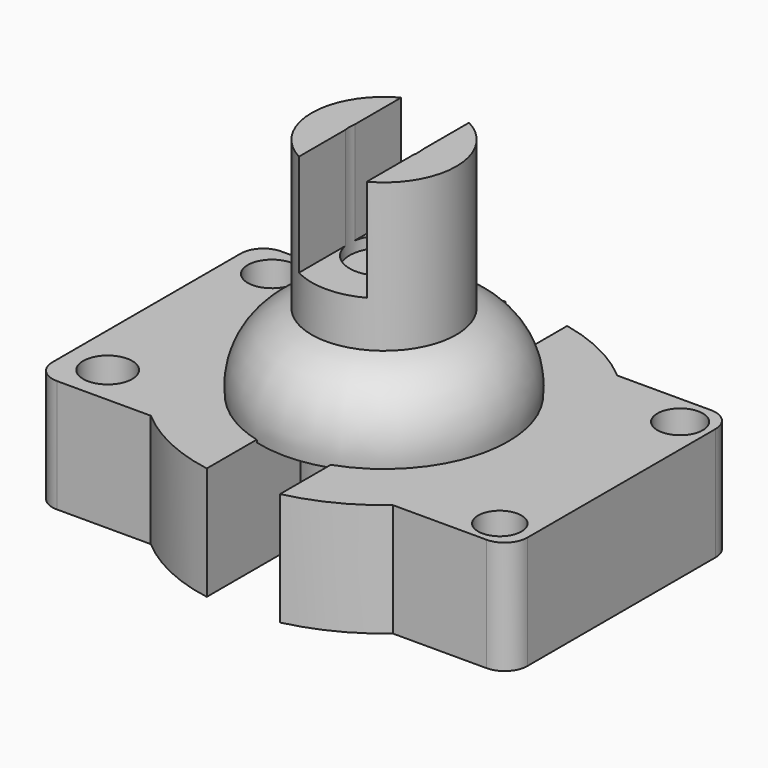
from build123d import *

# Parameters (mm, degrees)
F1_DEPTH       = 25.4
F2_R           = 5.4495134178
F2_R_2         = 5.5089125438
F3_DEPTH       = 25.4
F4_R           = 5.1025387704
F4_R_2         = 4.874193153
F5_DEPTH       = 25.4
F7_DEPTH       = 25.4
F9_DEPTH       = 25.4
F10_R          = 5.08
F15_R          = 7.7344411216
F16_DEPTH      = 25.4
F17_W          = 15.24
F17_H          = 33.801519665
F18_DEPTH      = 25.4
F18_DEPTH_BACK = 25.4


# Not quite as in the source:
# - a feature of the source that left no trace in its solid (it failed there, or was rolled back) is left out


with BuildPart() as f1:
    # F0 (on Top) → F1 (new body)
    with BuildSketch(Plane.XY):
        with BuildLine():
            Line((-53.3399991691, -31.5190926194), (-27.1817994649, -31.5190926194))
            ThreePointArc((-27.1817994649, -31.5190926194), (-41.6209493128, 0), (-27.1817994649, 31.5190926194))
            Line((-27.1817994649, 31.5190926194), (-53.3399991691, 31.5190926194))
            Line((-53.3399991691, 31.5190926194), (-53.3399991691, -31.5190926194))
        make_face()
        with BuildLine():
            Line((27.1817994649, -31.5190926194), (53.3399991691, -31.5190926194))
            Line((53.3399991691, -31.5190926194), (53.3399991691, 31.5190926194))
            Line((53.3399991691, 31.5190926194), (27.1817994649, 31.5190926194))
            ThreePointArc((27.1817994649, 31.5190926194), (37.8393691772, 17.3345193752), (41.6209493128, 0))
            ThreePointArc((41.6209493128, 0), (37.8393691772, -17.3345193752), (27.1817994649, -31.5190926194))
        make_face()
        with BuildLine():
            ThreePointArc((-27.1817994649, -31.5190926194), (0, -41.6209493128), (27.1817994649, -31.5190926194))
            Line((27.1817994649, -31.5190926194), (-27.1817994649, -31.5190926194))
        make_face()
        with BuildLine():
            Line((-27.1817994649, 31.5190926194), (27.1817994649, 31.5190926194))
            ThreePointArc((27.1817994649, 31.5190926194), (0, 41.6209493128), (-27.1817994649, 31.5190926194))
        make_face()
        with BuildLine():
            Line((-27.1817994649, -31.5190926194), (27.1817994649, -31.5190926194))
            ThreePointArc((27.1817994649, -31.5190926194), (37.8393691772, -17.3345193752), (41.6209493128, 0))
            ThreePointArc((41.6209493128, 0), (37.8393691772, 17.3345193752), (27.1817994649, 31.5190926194))
            Line((27.1817994649, 31.5190926194), (-27.1817994649, 31.5190926194))
            ThreePointArc((-27.1817994649, 31.5190926194), (-41.6209493128, 0), (-27.1817994649, -31.5190926194))
        make_face()
    extrude(amount=F1_DEPTH)

    # F2 (on face) → F3 (cut)
    with BuildSketch(Plane.XY.offset(25.4)):
        with Locations((-44.2123003304, 23.8175932318)):
            Circle(F2_R)
        with Locations((-43.9270585775, -22.6766318083)):
            Circle(F2_R_2)
    extrude(amount=-F3_DEPTH, mode=Mode.SUBTRACT)

    # F4 (on face) → F5 (cut)
    with BuildSketch(Plane.XY.offset(25.4)):
        with Locations((46.7794649303, 24.6733147651)):
            Circle(F4_R)
        with Locations((46.2089851499, -25.2437964082)):
            Circle(F4_R_2)
    extrude(amount=-F5_DEPTH, mode=Mode.SUBTRACT)

    # F6 (on face) → F7 (cut)
    with BuildSketch(Plane.XY.offset(25.4)):
        with BuildLine():
            Line((-6.9852194627, -11.5522462875), (-6.9852194627, -41.0305999317))
            Line((-6.9852194627, -41.0305999317), (6.9852194627, -41.0305999317))
            ThreePointArc((6.9852194627, -41.0305999317), (8.0592339465, -40.8332238489), (9.1277007014, -40.6077394299))
            Line((9.1277007014, -40.6077394299), (9.1277007014, -11.5522462875))
            Line((9.1277007014, -11.5522462875), (-6.9852194627, -11.5522462875))
        make_face()
        with BuildLine():
            Line((6.9852194627, -41.0305999317), (-6.9852194627, -41.0305999317))
            ThreePointArc((-6.9852194627, -41.0305999317), (0, -41.6209493128), (6.9852194627, -41.0305999317))
        make_face()
        with BuildLine():
            Line((5.7398033244, 41.2232710917), (-5.7398033244, 41.2232710917))
            Line((-5.7398033244, 41.2232710917), (-5.7398033244, 11.2670054659))
            Line((-5.7398033244, 11.2670054659), (8.5572190583, 11.2670054659))
            Line((8.5572190583, 11.2670054659), (8.5572190583, 40.7317741289))
            ThreePointArc((8.5572190583, 40.7317741289), (7.1527340625, 41.0017294407), (5.7398033244, 41.2232710917))
        make_face()
    extrude(amount=-F7_DEPTH, mode=Mode.SUBTRACT)

    # F9 (cut): a face of the model
    f9_faces = [f1.faces().sort_by_distance(p)[0] for p in [
        (0, 41.2232710917, 12.7),
    ]]
    extrude(f9_faces, amount=-F9_DEPTH, mode=Mode.SUBTRACT)

    # F10
    f10_edges = [f1.edges().sort_by_distance(p)[0] for p in [
        (53.339999, -31.519093, 12.7),
        (53.339999, 31.519093, 12.7),
        (-53.339999, -31.519093, 12.7),
        (-53.339999, 31.519093, 12.7),
    ]]
    fillet(f10_edges, radius=F10_R)

    # F11 (on Front) → F12 (revolve)
    with BuildSketch(Plane.XZ):
        Polygon((-16.2587165833, 0), (0, 0), (0, 76.0166272521), (-16.2587165833, 76.0166272521), (-16.2587165833, 42.7147820592), (-16.2587165833, 24.7446224093), align=None)
    revolve(axis=Axis((0, 0, 38.0083136261), (0, 0, 1)))

    # F11 (on Front) → F13 (revolve)
    with BuildSketch(Plane.XZ):
        Polygon((-16.2587165833, 0), (0, 0), (0, 76.0166272521), (-16.2587165833, 76.0166272521), (-16.2587165833, 42.7147820592), (-16.2587165833, 24.7446224093), align=None)
        with BuildLine():
            Line((-27.8109610081, 24.7446224093), (-16.2587165833, 24.7446224093))
            Line((-16.2587165833, 24.7446224093), (-16.2587165833, 42.7147820592))
            ThreePointArc((-16.2587165833, 42.7147820592), (-25.501298739, 35.958140564), (-27.8109610081, 24.7446224093))
        make_face()
    revolve(axis=Axis((0, 0, 76.0166272521), (0, 0, -1)))

    # F15 (on face) → F16 (cut)
    with BuildSketch(Plane.XY.offset(76.0166272521)):
        Circle(F15_R)
    extrude(amount=-F16_DEPTH, mode=Mode.SUBTRACT)

    # F17 (on Front) → F18 (cut, two sides)
    with BuildSketch(Plane.XZ) as f18_sk:
        with Locations((0, 69.9550167755)):
            Rectangle(F17_W, F17_H)
    extrude(amount=-F18_DEPTH, mode=Mode.SUBTRACT)
    extrude(f18_sk.sketch, amount=F18_DEPTH_BACK, mode=Mode.SUBTRACT)


solid = f1.part
